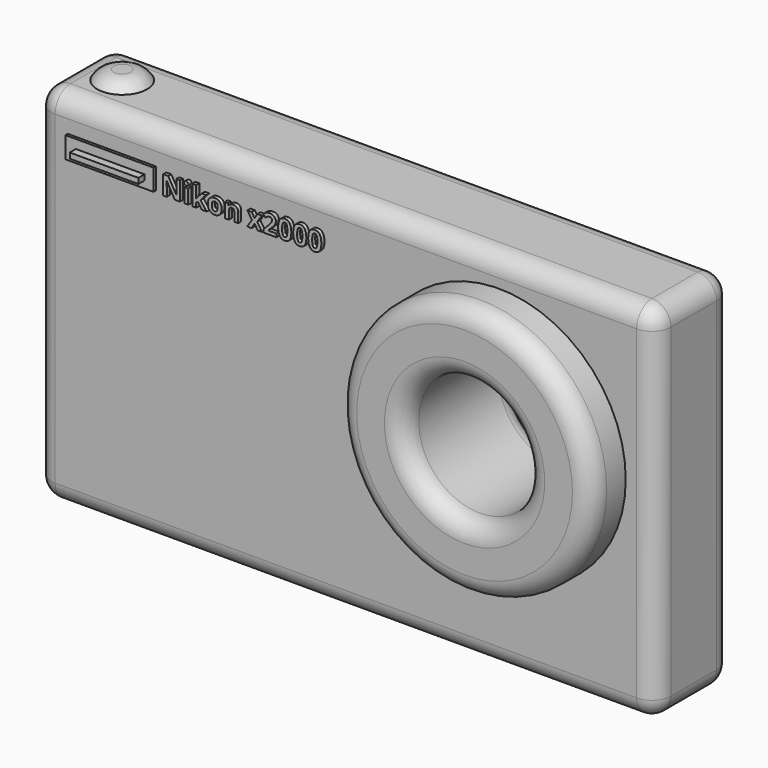
from build123d import *

# Parameters (mm, degrees)
F0_W          = 165.3469055891
F0_H          = 96.8583319336
F1_DEPTH      = 25.4
F2_R          = 33.8706825457
F3_DEPTH      = 11.43
F4_R          = 16.311421591
F5_DEPTH      = 36.831
F6_R          = 5.08
F7_R          = 5.08
F8_T1_DEPTH   = 15.24
F8_S5_W       = 5.08
F8_S5_H       = 5.08
F8_T6_DEPTH   = 5.08
F8_S11_W      = 5.08
F8_S11_H      = 5.08
F8_T12_DEPTH  = 5.08
F8_S17_W      = 5.08
F8_S17_H      = 5.08
F8_T18_DEPTH  = 5.08
F8_S23_W      = 5.08
F8_S23_H      = 5.08
F8_T24_DEPTH  = 5.08
F8_S29_W      = 5.08
F8_S29_H      = 5.08
F8_T30_DEPTH  = 5.08
F8_S35_W      = 5.08
F8_S35_H      = 5.08
F8_T36_DEPTH  = 5.08
F8_S41_W      = 5.08
F8_S41_H      = 5.08
F8_T42_DEPTH  = 5.08
F8_S47_W      = 5.08
F8_S47_H      = 5.08
F8_T48_DEPTH  = 5.08
F9_R          = 6.6528395831
F10_DEPTH     = 2.54
F12_W         = 83.3050990477
F12_H         = 71.2683950551
F13_DEPTH     = 1.27
F14_W         = 23.4931632876
F14_H         = 5.687572062
F15_DEPTH     = 0.762
F16_TEXT_SIZE = 7.0214581986
F17_DEPTH     = 1.016
F18_W         = 18.3176621795
F18_H         = 1.4528334141
F19_DEPTH     = 2.032


# Not quite as in the source:
# - a fillet or chamfer that OpenCascade refuses, or shapes differently, is made with other operations: its cross-section is extruded or revolved along the edge and cut away or added
# - Text() gives the source's letters only with a copy of the font that has no kerning and outlines rounded to 1/6400 em; it was checked with that copy


with BuildPart() as f1:
    # F0 (on Front) → F1 (new body)
    with BuildSketch(Plane.XZ):
        with Locations((2.7223452926, 27.0802108571)):
            Rectangle(F0_W, F0_H)
    extrude(amount=F1_DEPTH)

    # F2 (on face) → F3 (join)
    with BuildSketch(Plane.XZ.offset(25.4)):
        with Locations((43.5324683785, 34.0743400156)):
            Circle(F2_R)
    extrude(amount=F3_DEPTH)

    # F4 (on face) → F5 (cut, through all)
    with BuildSketch(Plane.XZ.offset(36.83)):
        with Locations((43.5324683785, 34.0743400156)):
            Circle(F4_R)
    extrude(amount=-F5_DEPTH, mode=Mode.SUBTRACT)

    # F6
    f6_edges = [f1.edges().sort_by_distance(p)[0] for p in [
        (9.661786, -36.83, 34.07434),
        (27.221047, -36.83, 34.07434),
        (2.722345, -25.4, 75.509377),
        (85.395798, -25.4, 27.080211),
        (-79.951108, -25.4, 27.080211),
        (2.722345, -25.4, -21.348955),
    ]]
    fillet(f6_edges, radius=F6_R)

    # F7
    f7_edges = [f1.edges().sort_by_distance(p)[0] for p in [
        (27.221047, 0, 34.07434),
        (85.395798, 0, 27.080211),
        (2.722345, 0, 75.509377),
        (2.722345, 0, -21.348955),
        (-79.951108, 0, 27.080211),
    ]]
    fillet(f7_edges, radius=F7_R)

    # F8: fillet of radius 5.08 on 4 edges, made by hand

    # F8_s2 → F8_t1 (cut)
    with BuildSketch(Plane.XZ.offset(5.08)):
        with BuildLine():
            ThreePointArc((80.3157980871, 75.5093768239), (83.9079005355, 74.0214792723), (85.3957980871, 70.4293768239))
            Line((85.3957980871, 70.4293768239), (85.3957980871, 75.5093768239))
            Line((85.3957980871, 75.5093768239), (80.3157980871, 75.5093768239))
        make_face()
        with BuildLine():
            ThreePointArc((85.3957980871, -16.2689551097), (83.9079005355, -19.8610575581), (80.3157980871, -21.3489551097))
            Line((80.3157980871, -21.3489551097), (85.3957980871, -21.3489551097))
            Line((85.3957980871, -21.3489551097), (85.3957980871, -16.2689551097))
        make_face()
        with BuildLine():
            ThreePointArc((-79.951107502, -16.2689551097), (-78.4632099504, -19.8610575581), (-74.871107502, -21.3489551097))
            Line((-74.871107502, -21.3489551097), (-79.951107502, -21.3489551097))
            Line((-79.951107502, -21.3489551097), (-79.951107502, -16.2689551097))
        make_face()
        with BuildLine():
            ThreePointArc((-74.871107502, 75.5093768239), (-78.4632099504, 74.0214792723), (-79.951107502, 70.4293768239))
            Line((-79.951107502, 70.4293768239), (-79.951107502, 75.5093768239))
            Line((-79.951107502, 75.5093768239), (-74.871107502, 75.5093768239))
        make_face()
    extrude(amount=F8_T1_DEPTH, mode=Mode.SUBTRACT)


with BuildPart() as f8_tool4:
    # F8_s5 → F8_t6 (new body)
    with BuildSketch(Plane.XY.offset(70.4293768239)):
        with Locations((-77.411107502, -2.54)):
            Rectangle(F8_S5_W, F8_S5_H)
    extrude(amount=F8_T6_DEPTH)

    # F8_s7 → F8_t8 (revolve, cut)
    with BuildSketch(Plane(origin=(-74.871107502, -5.08, 70.4293768239), x_dir=(0.7071067812, -0.7071067812, 0), z_dir=(-0.7071067812, -0.7071067812, 0))):
        with BuildLine():
            ThreePointArc((0, -5.08), (5.08, 0), (0, 5.08))
            Line((0, 5.08), (0, -5.08))
        make_face()
    revolve(axis=Axis((-74.871107502, -5.08, 70.4293768239), (0, 0, 1)), mode=Mode.SUBTRACT)


with BuildPart() as f1_1:
    add(f1.part)

    # F8_t3: cut F8_tool4
    add(f8_tool4.part, mode=Mode.SUBTRACT)


with BuildPart() as f8_tool10:
    # F8_s11 → F8_t12 (new body)
    with BuildSketch(Plane.XY.offset(70.4293768239)):
        with Locations((-77.411107502, -22.86)):
            Rectangle(F8_S11_W, F8_S11_H)
    extrude(amount=F8_T12_DEPTH)

    # F8_s13 → F8_t14 (revolve, cut)
    with BuildSketch(Plane(origin=(-74.871107502, -20.32, 70.4293768239), x_dir=(0.7071067812, 0.7071067812, 0), z_dir=(0.7071067812, -0.7071067812, 0))):
        with BuildLine():
            ThreePointArc((0, -5.08), (5.08, 0), (0, 5.08))
            Line((0, 5.08), (0, -5.08))
        make_face()
    revolve(axis=Axis((-74.871107502, -20.32, 70.4293768239), (0, 0, 1)), mode=Mode.SUBTRACT)


with BuildPart() as f1_2:
    add(f1_1.part)

    # F8_t9: cut F8_tool10
    add(f8_tool10.part, mode=Mode.SUBTRACT)


with BuildPart() as f8_tool16:
    # F8_s17 → F8_t18 (new body)
    with BuildSketch(Plane.YZ.offset(-74.871107502)):
        with Locations((-2.54, -18.8089551097)):
            Rectangle(F8_S17_W, F8_S17_H)
    extrude(amount=-F8_T18_DEPTH)

    # F8_s19 → F8_t20 (revolve, cut)
    with BuildSketch(Plane(origin=(-74.871107502, -5.08, -16.2689551097), x_dir=(0, -0.7071067812, 0.7071067812), z_dir=(0, -0.7071067812, -0.7071067812))):
        with BuildLine():
            ThreePointArc((0, -5.08), (5.08, 0), (0, 5.08))
            Line((0, 5.08), (0, -5.08))
        make_face()
    revolve(axis=Axis((-74.871107502, -5.08, -16.2689551097), (-1, 0, 0)), mode=Mode.SUBTRACT)


with BuildPart() as f1_3:
    add(f1_2.part)

    # F8_t15: cut F8_tool16
    add(f8_tool16.part, mode=Mode.SUBTRACT)


with BuildPart() as f8_tool22:
    # F8_s23 → F8_t24 (new body)
    with BuildSketch(Plane.YZ.offset(-74.871107502)):
        with Locations((-22.86, -18.8089551097)):
            Rectangle(F8_S23_W, F8_S23_H)
    extrude(amount=-F8_T24_DEPTH)

    # F8_s25 → F8_t26 (revolve, cut)
    with BuildSketch(Plane(origin=(-74.871107502, -20.32, -16.2689551097), x_dir=(0, 0.7071067812, 0.7071067812), z_dir=(0, -0.7071067812, 0.7071067812))):
        with BuildLine():
            ThreePointArc((0, -5.08), (5.08, 0), (0, 5.08))
            Line((0, 5.08), (0, -5.08))
        make_face()
    revolve(axis=Axis((-74.871107502, -20.32, -16.2689551097), (-1, 0, 0)), mode=Mode.SUBTRACT)


with BuildPart() as f1_4:
    add(f1_3.part)

    # F8_t21: cut F8_tool22
    add(f8_tool22.part, mode=Mode.SUBTRACT)


with BuildPart() as f8_tool28:
    # F8_s29 → F8_t30 (new body)
    with BuildSketch(Plane.YZ.offset(80.3157980871)):
        with Locations((-2.54, -18.8089551097)):
            Rectangle(F8_S29_W, F8_S29_H)
    extrude(amount=F8_T30_DEPTH)

    # F8_s31 → F8_t32 (revolve, cut)
    with BuildSketch(Plane(origin=(80.3157980871, -5.08, -16.2689551097), x_dir=(0, -0.7071067812, 0.7071067812), z_dir=(0, 0.7071067812, 0.7071067812))):
        with BuildLine():
            ThreePointArc((0, -5.08), (5.08, 0), (0, 5.08))
            Line((0, 5.08), (0, -5.08))
        make_face()
    revolve(axis=Axis((80.3157980871, -5.08, -16.2689551097), (1, 0, 0)), mode=Mode.SUBTRACT)


with BuildPart() as f1_5:
    add(f1_4.part)

    # F8_t27: cut F8_tool28
    add(f8_tool28.part, mode=Mode.SUBTRACT)


with BuildPart() as f8_tool34:
    # F8_s35 → F8_t36 (new body)
    with BuildSketch(Plane.YZ.offset(80.3157980871)):
        with Locations((-22.86, -18.8089551097)):
            Rectangle(F8_S35_W, F8_S35_H)
    extrude(amount=F8_T36_DEPTH)

    # F8_s37 → F8_t38 (revolve, cut)
    with BuildSketch(Plane(origin=(80.3157980871, -20.32, -16.2689551097), x_dir=(0, 0.7071067812, 0.7071067812), z_dir=(0, 0.7071067812, -0.7071067812))):
        with BuildLine():
            ThreePointArc((0, -5.08), (5.08, 0), (0, 5.08))
            Line((0, 5.08), (0, -5.08))
        make_face()
    revolve(axis=Axis((80.3157980871, -20.32, -16.2689551097), (1, 0, 0)), mode=Mode.SUBTRACT)


with BuildPart() as f1_6:
    add(f1_5.part)

    # F8_t33: cut F8_tool34
    add(f8_tool34.part, mode=Mode.SUBTRACT)


with BuildPart() as f8_tool40:
    # F8_s41 → F8_t42 (new body)
    with BuildSketch(Plane.XY.offset(70.4293768239)):
        with Locations((82.8557980871, -2.54)):
            Rectangle(F8_S41_W, F8_S41_H)
    extrude(amount=F8_T42_DEPTH)

    # F8_s43 → F8_t44 (revolve, cut)
    with BuildSketch(Plane(origin=(80.3157980871, -5.08, 70.4293768239), x_dir=(-0.7071067812, -0.7071067812, 0), z_dir=(-0.7071067812, 0.7071067812, 0))):
        with BuildLine():
            ThreePointArc((0, -5.08), (5.08, 0), (0, 5.08))
            Line((0, 5.08), (0, -5.08))
        make_face()
    revolve(axis=Axis((80.3157980871, -5.08, 70.4293768239), (0, 0, 1)), mode=Mode.SUBTRACT)


with BuildPart() as f1_7:
    add(f1_6.part)

    # F8_t39: cut F8_tool40
    add(f8_tool40.part, mode=Mode.SUBTRACT)


with BuildPart() as f8_tool46:
    # F8_s47 → F8_t48 (new body)
    with BuildSketch(Plane.XY.offset(70.4293768239)):
        with Locations((82.8557980871, -22.86)):
            Rectangle(F8_S47_W, F8_S47_H)
    extrude(amount=F8_T48_DEPTH)

    # F8_s49 → F8_t50 (revolve, cut)
    with BuildSketch(Plane(origin=(80.3157980871, -20.32, 70.4293768239), x_dir=(-0.7071067812, 0.7071067812, 0), z_dir=(0.7071067812, 0.7071067812, 0))):
        with BuildLine():
            ThreePointArc((0, -5.08), (5.08, 0), (0, 5.08))
            Line((0, 5.08), (0, -5.08))
        make_face()
    revolve(axis=Axis((80.3157980871, -20.32, 70.4293768239), (0, 0, 1)), mode=Mode.SUBTRACT)


with BuildPart() as f1_8:
    add(f1_7.part)

    # F8_t45: cut F8_tool46
    add(f8_tool46.part, mode=Mode.SUBTRACT)

    # F9 (on face) → F10 (join)
    with BuildSketch(Plane.XY.offset(75.5093768239)):
        with Locations((-67.4593821168, -12.3100178316)):
            Circle(F9_R)
    extrude(amount=F10_DEPTH)

    # F11: fillet of radius 5.08 on 1 edges, made by hand

    # F11_s1 → F11_t2 (revolve, cut)
    with BuildSketch(Plane.XZ.offset(12.3100178316)):
        with BuildLine():
            ThreePointArc((-60.8065425337, 75.5093768239), (-62.6659515849, 77.3687858751), (-65.2059515849, 78.0493768239))
            Line((-65.2059515849, 78.0493768239), (-60.8065425337, 78.0493768239))
            Line((-60.8065425337, 78.0493768239), (-60.8065425337, 75.5093768239))
        make_face()
    revolve(axis=Axis((-67.4593821168, -12.3100178316, 78.0493768239), (0, 0, 1)), mode=Mode.SUBTRACT)

    # F12 (on face) → F13 (join)
    with BuildSketch(Plane(origin=(0, 0, 0), x_dir=(-1, 0, 0), z_dir=(0, 1, 0))):
        with Locations((27.2998395376, 28.1355527695)):
            Rectangle(F12_W, F12_H)
    extrude(amount=F13_DEPTH)

    # F14 (on face) → F15 (join)
    with BuildSketch(Plane.XZ.offset(25.4)):
        with Locations((-59.7696863115, 64.0424676239)):
            Rectangle(F14_W, F14_H)
    extrude(amount=F15_DEPTH)

    # F16 (on face) → F17 (join)
    with BuildSketch(Plane.XZ.offset(25.4)):
        with Locations((-45.8618365228, 61.3508448005)):
            Text('Nikon x2000', F16_TEXT_SIZE, font='Open Sans', font_style=FontStyle.BOLD, text_align=(TextAlign.LEFT, TextAlign.BOTTOM))
    extrude(amount=F17_DEPTH)

    # F18 (on face) → F19 (join)
    with BuildSketch(Plane.XZ.offset(26.162)):
        with Locations((-59.5842413604, 63.8052597642)):
            Rectangle(F18_W, F18_H)
    extrude(amount=F19_DEPTH)


solid = f1_8.part
